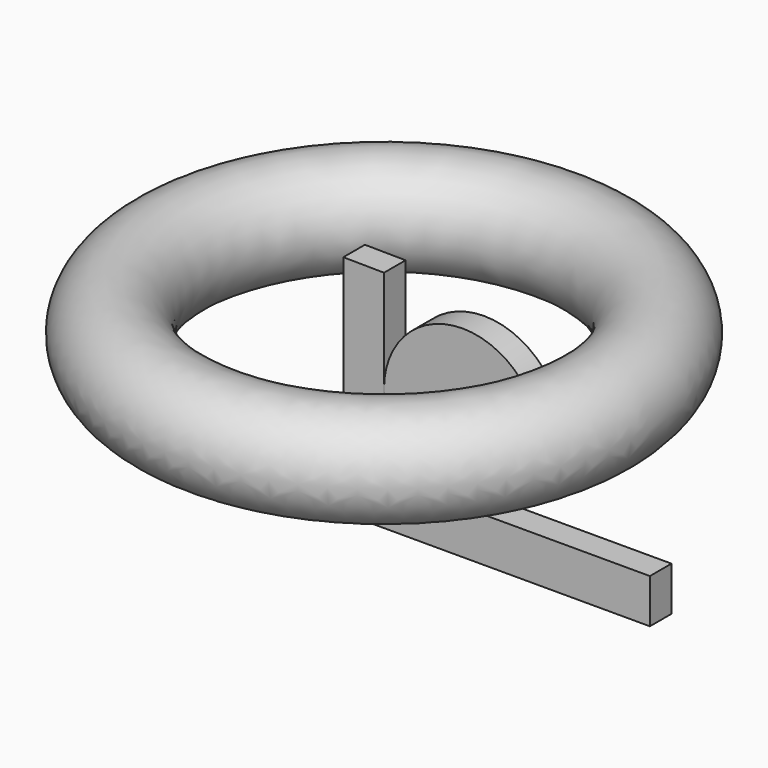
from build123d import *

# Parameters (mm, degrees)
F1_DEPTH = 25.4
F3_DEPTH = 25.4
F2_R     = 47.9820834299


# Not quite as in the source:
# - the program builds the solid bodies; features that only make, move or delete a surface that nothing else refers to are left out


with BuildPart() as f1:
    # F0 (on Front) → F1 (new body)
    with BuildSketch(Plane.XZ):
        Polygon((-92.7426367998, 115.0774434209), (-131.0308873653, 115.502871573), (-131.0308873653, -96.7841818929), (157.8326672316, -96.7841818929), (157.8326672316, -55.0925396383), (-92.7426367998, -55.0925396383), align=None)
    extrude(amount=F1_DEPTH)

    # F2 (on Front) → F3 (join)
    with BuildSketch(Plane.XZ):
        with BuildLine():
            ThreePointArc((-92.7426367998, 18.9314040204), (-71.0615257881, -33.4114285499), (-18.7186932496, -55.0925396383))
            ThreePointArc((-18.7186932496, -55.0925396383), (33.6241389941, -33.4114285331), (55.305249989, 18.9314037561))
            ThreePointArc((55.305249989, 18.9314037561), (-18.7186932733, 92.9553471506), (-92.7426367998, 18.9314040204))
        make_face()
    extrude(amount=F3_DEPTH)


with BuildPart() as f5:
    # F2 (on Front) → F5 (revolve)
    with BuildSketch(Plane.XZ):
        with Locations((106.7868769169, 65.1014372706)):
            Circle(F2_R)
    revolve(axis=Axis((-92.7426367998, -25.4, 67.0044234123), (0, 0, 1)))


solid = Compound([f1.part, f5.part])
